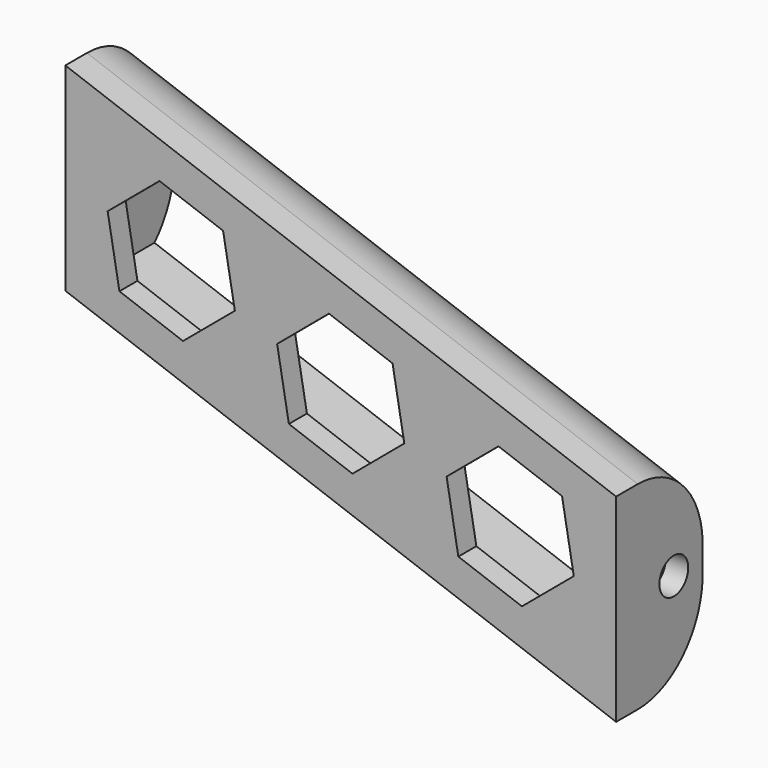
from build123d import *

# Parameters (mm, degrees)
F1_DEPTH    = 12
F2_T        = -2.5
F4_D        = 4
F4_DEPTH    = 6
F4_TIP      = 1.2017212381
F6_D        = 4
F6_DEPTH    = 6
F6_TIP      = 1.2017212381
F8_DEPTH    = 25
F9_T1_DEPTH = 110
F9_T3_DEPTH = 110


# Not quite as in the source:
# - a fillet or chamfer that OpenCascade refuses, or shapes differently, is made with other operations: its cross-section is extruded or revolved along the edge and cut away or added


with BuildPart() as f1:
    # F0 (on Front) → F1 (new body)
    with BuildSketch(Plane.XZ):
        Polygon((18.7692175617, 10.3012606697), (-42.3108027894, 32.5325699859), (-42.3108027894, 10.5325699859), (18.7692175617, -11.6987393303), align=None)
    extrude(amount=-F1_DEPTH)

    # F2
    f2_openings = [f1.faces().sort_by_distance(p)[0] for p in [
        (-11.770793, 12, 10.416915),
    ]]
    offset(amount=F2_T, openings=f2_openings)

    # F4
    with Locations(Plane.YZ.offset(18.7692175617)):
        with Locations((8, -0.6987393303)):
            Hole(F4_D / 2, depth=F4_DEPTH)
            with Locations((0, 0, -(F4_DEPTH + F4_TIP / 2))):  # 118° drill point
                Cone(0, F4_D / 2, F4_TIP, mode=Mode.SUBTRACT)

    # F6
    with Locations(Plane(origin=(-42.3108027894, 0, 0), x_dir=(0, -1, 0), z_dir=(-1, 0, 0))):
        with Locations((-8, 21.5325699859)):
            Hole(F6_D / 2, depth=F6_DEPTH)
            with Locations((0, 0, -(F6_DEPTH + F6_TIP / 2))):  # 118° drill point
                Cone(0, F6_D / 2, F6_TIP, mode=Mode.SUBTRACT)

    # F7 (on face) → F8 (cut)
    with BuildSketch(Plane(origin=(0, 2.5, 0), x_dir=(-1, 0, 0), z_dir=(0, 1, 0))):
        Polygon((-1.2734722511, -1.247964332), (0.0298534365, 6.1435629449), (-5.7197341143, 10.9680397382), (-12.7726473527, 8.4009892546), (-14.0759730402, 1.0094619776), (-8.3263854894, -3.8150148157), align=None)
        Polygon((10.4674669263, 3.0253880509), (17.5203801646, 5.5924385345), (18.8237058522, 12.9839658114), (13.0741183014, 17.8084426047), (6.021205063, 15.2413921211), (4.7178793755, 7.8498648442), align=None)
        Polygon((29.261319342, 9.8657909174), (36.3142325804, 12.432841401), (37.6175582679, 19.8243686779), (31.8679707171, 24.6488454712), (24.8150574788, 22.0817949876), (23.5117317912, 14.6902677107), align=None)
    extrude(amount=-F8_DEPTH, mode=Mode.SUBTRACT)

    # F9: fillet of radius 9 on 2 edges, made by hand

    # F9_s2 → F9_t1 (cut)
    with BuildSketch(Plane(origin=(34.4059587946, 0, -12.5227448826), x_dir=(0, 1, 0), z_dir=(-0.9396926208, 0, 0.3420201433))):
        with BuildLine():
            ThreePointArc((3, -16.0994691167), (9.3639610307, -13.4634301474), (12, -7.0994691167))
            Line((12, -7.0994691167), (12, -16.0994691167))
            Line((12, -16.0994691167), (3, -16.0994691167))
        make_face()
    extrude(amount=F9_T1_DEPTH, mode=Mode.SUBTRACT)

    # F9_s4 → F9_t3 (cut)
    with BuildSketch(Plane(origin=(-61.8895657853, 0, 22.5259597575), x_dir=(0, 1, 0), z_dir=(0.9396926208, 0, -0.3420201433))):
        with BuildLine():
            ThreePointArc((12, 4.4262314594), (9.3639610307, -1.9377295713), (3, -4.5737685406))
            Line((3, -4.5737685406), (12, -4.5737685406))
            Line((12, -4.5737685406), (12, 4.4262314594))
        make_face()
    extrude(amount=F9_T3_DEPTH, mode=Mode.SUBTRACT)


solid = f1.part
